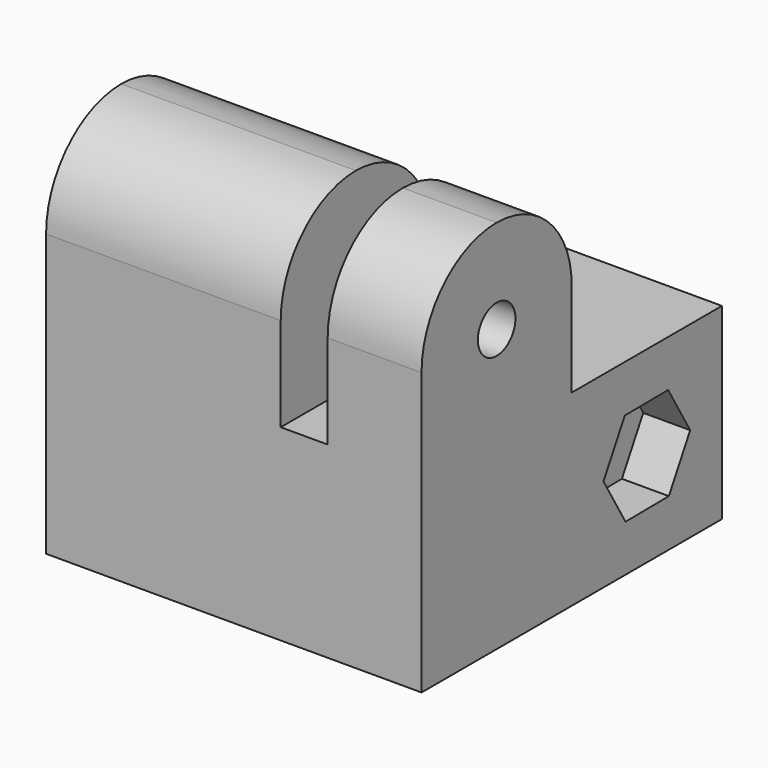
from build123d import *

# Parameters (mm, degrees)
F0_W      = 50.8
F0_H      = 50.8
F1_DEPTH  = 25.4
F3_DEPTH  = 25.4
F4_R      = 3.175
F5_DEPTH  = 50.801
F6_W      = 6.35
F6_H      = 29.9948125449
F6_H_2    = 12.7
F7_DEPTH  = 50.801
F8_R      = 3.175
F9_DEPTH  = 6.35
F10_DEPTH = 6.35
F11_DEPTH = 1.5875


# Not quite as in the source:
# - a feature names something its author has since deleted; it is built from what else it names


with BuildPart() as f1:
    # F0 (on Front) → F1 (new body, symmetric)
    with BuildSketch(Plane.XZ):
        with Locations((-1.9110422581, 1.9712704602)):
            Rectangle(F0_W, F0_H)
    extrude(amount=F1_DEPTH, both=True)

    # F2 (on face) → F3 (cut)
    with BuildSketch(Plane(origin=(0, 0, -23.4287295398), x_dir=(1, 0, 0), z_dir=(0, 0, -1))):
        with BuildLine():
            Line((-6.6735422581, -6.4520295568), (-6.6735422581, 0))
            ThreePointArc((-6.6735422581, 0), (-8.2610422581, 12.4983610621), (-9.8485422581, 0))
            Line((-9.8485422581, 0), (-9.8485422581, -6.4520295568))
            ThreePointArc((-9.8485422581, -6.4520295568), (-8.2610422581, -6.5516389379), (-6.6735422581, -6.4520295568))
        make_face()
        with BuildLine():
            Line((-6.6735422581, -25.4), (-6.6735422581, -6.4520295568))
            ThreePointArc((-6.6735422581, -6.4520295568), (-8.2610422581, -6.5516389379), (-9.8485422581, -6.4520295568))
            Line((-9.8485422581, -6.4520295568), (-9.8485422581, -25.4))
            Line((-9.8485422581, -25.4), (-6.6735422581, -25.4))
        make_face()
    extrude(amount=-F3_DEPTH, mode=Mode.SUBTRACT)

    # F4 (on face) → F5 (cut, through all)
    with BuildSketch(Plane.YZ.offset(23.4889577419)):
        with BuildLine():
            Line((-25.4, 27.3712704602), (-25.4, 14.6712704602))
            ThreePointArc((-25.4, 14.6712704602), (-21.6802561342, 23.6515265681), (-12.7000000372, 27.3712704602))
            Line((-12.7000000372, 27.3712704602), (-25.4, 27.3712704602))
        make_face()
        with BuildLine():
            Line((0, 14.6712704602), (0, 1.9712704602))
            Line((0, 1.9712704602), (25.4, 1.9712704602))
            Line((25.4, 1.9712704602), (25.4, 27.3712704602))
            Line((25.4, 27.3712704602), (-12.7000000372, 27.3712704602))
            ThreePointArc((-12.7000000372, 27.3712704602), (-3.7197438921, 23.6515265944), (0, 14.6712704602))
        make_face()
        with Locations((-12.7, 14.6712704602)):
            Circle(F4_R)
        with Locations((12.7, -10.7287295398)):
            Circle(F4_R)
    extrude(amount=-F5_DEPTH, mode=Mode.SUBTRACT)

    # F6 (on face) → F7 (cut, through all)
    with BuildSketch(Plane.XZ.offset(25.4)):
        with Locations((7.6139577419, 29.6686767327)):
            Rectangle(F6_W, F6_H)
        with Locations((7.6139577419, 8.3212704602)):
            Rectangle(F6_W, F6_H_2)
    extrude(amount=-F7_DEPTH, mode=Mode.SUBTRACT)

    # F8 (on face) → F9 (cut)
    with BuildSketch(Plane(origin=(-27.3110422581, 0, 0), x_dir=(0, -1, 0), z_dir=(-1, 0, 0))):
        Polygon((9.0338257906, 21.0212704602), (5.3676515813, 14.6712704602), (9.0338257906, 8.3212704602), (16.3661742094, 8.3212704602), (20.0323484187, 14.6712704602), (16.3661742094, 21.0212704602), align=None)
        with Locations((12.7, 14.6712704602)):
            Circle(F8_R, mode=Mode.SUBTRACT)
    extrude(amount=-F9_DEPTH, mode=Mode.SUBTRACT)

    # F4 (on face) → F10 (cut)
    with BuildSketch(Plane.YZ.offset(23.4889577419)):
        Polygon((16.4270880107, -17.0431692056), (20.0320091667, -10.6581964733), (16.3049211559, -4.3437568074), (8.9729119893, -4.414289874), (5.3679908333, -10.7992626063), (9.0950788441, -17.1137022722), align=None)
        with Locations((12.7, -10.7287295398)):
            Circle(F4_R, mode=Mode.SUBTRACT)
    extrude(amount=-F10_DEPTH, mode=Mode.SUBTRACT)

    # F2 (on face) → F11 (cut)
    with BuildSketch(Plane(origin=(0, 0, -23.4287295398), x_dir=(1, 0, 0), z_dir=(0, 0, -1))):
        with BuildLine():
            ThreePointArc((-9.8485422581, 0), (-8.2610422581, 12.4983610621), (-6.6735422581, 0))
            Line((-6.6735422581, 0), (-6.6735422581, -6.4520295568))
            ThreePointArc((-6.6735422581, -6.4520295568), (1.2639577419, -2.2518993505), (4.4389577419, 6.1483610621))
            ThreePointArc((4.4389577419, 6.1483610621), (-16.6613026708, 15.6733610621), (-9.8485422581, -6.4520295568))
            Line((-9.8485422581, -6.4520295568), (-9.8485422581, 0))
        make_face()
    extrude(amount=-F11_DEPTH, mode=Mode.SUBTRACT)


solid = f1.part
